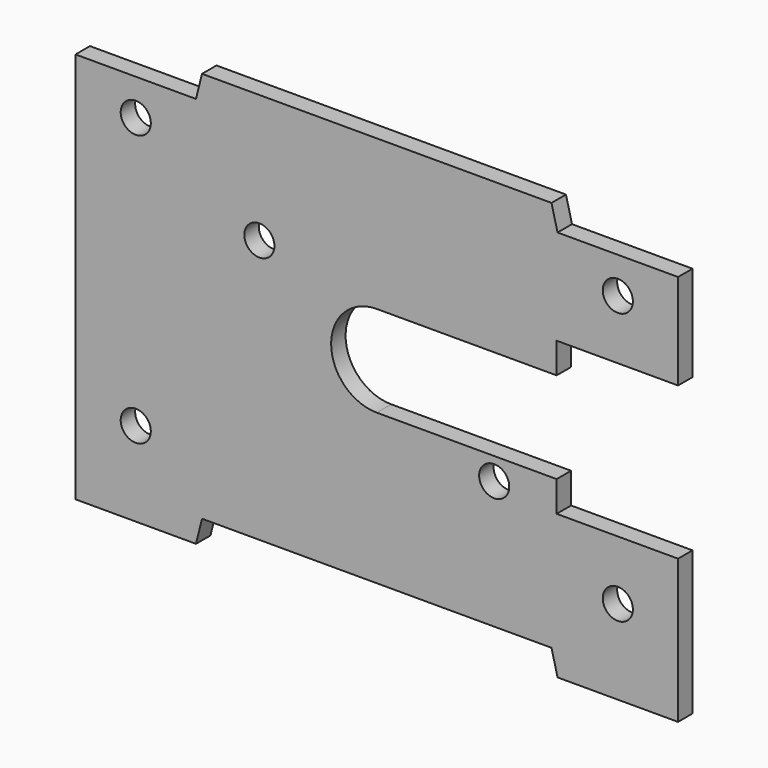
from build123d import *

# Parameters (mm, degrees)
F0_R     = 5
F0_W     = 40
F0_H     = 8
F1_DEPTH = 6


# Not quite as in the source:
# - a feature names something its author has since deleted; it is built from what else it names


with BuildPart() as f1:
    # F0 (on Front) → F1 (new body)
    with BuildSketch(Plane.XZ):
        with BuildLine():
            Line((0, 122), (0, 0))
            Line((0, 0), (40, 0))
            Line((40, 0), (42, 0))
            Line((42, 0), (158, 0))
            Line((158, 0), (160, 0))
            Line((160, 0), (200, 0))
            Line((200, 0), (200, 39.7))
            Line((200, 39.7), (159.7, 39.7))
            Line((159.7, 39.7), (159.7, 49.85))
            Line((159.7, 49.85), (126.2405697347, 49.85))
            Line((126.2405697347, 49.85), (100, 49.85))
            ThreePointArc((100, 49.85), (86.8797151327, 57.425), (86.8797151327, 72.575))
            ThreePointArc((86.8797151327, 72.575), (92.425, 78.1202848673), (100, 80.15))
            Line((100, 80.15), (159.7, 80.15))
            Line((159.7, 80.15), (159.7, 90.3))
            Line((159.7, 90.3), (200, 90.3))
            Line((200, 90.3), (200, 122))
            Line((200, 122), (160, 122))
            Line((160, 122), (158, 130))
            Line((158, 130), (42, 130))
            Line((42, 130), (40, 122))
            Line((40, 122), (0, 122))
        make_face()
        with Locations((20, 20)):
            Circle(F0_R, mode=Mode.SUBTRACT)
        with Locations((180, 20)):
            Circle(F0_R, mode=Mode.SUBTRACT)
        with BuildLine():
            ThreePointArc((143.9711431703, 42.5), (137.6770479448, 37.6703708686), (134.6410161514, 45))
            ThreePointArc((134.6410161514, 45), (140.2652383958, 47.3296291314), (143.9711431703, 42.5))
        make_face(mode=Mode.SUBTRACT)
        with BuildLine():
            ThreePointArc((66.0288568297, 87.5), (65.8584859611, 86.2059047745), (65.3589838486, 85))
            ThreePointArc((65.3589838486, 85), (56.1992276983, 88.7940952255), (66.0288568297, 87.5))
        make_face(mode=Mode.SUBTRACT)
        with Locations((20, 110)):
            Circle(F0_R, mode=Mode.SUBTRACT)
        with Locations((180, 110)):
            Circle(F0_R, mode=Mode.SUBTRACT)
        with Locations((20, -4)):
            Rectangle(F0_W, F0_H)
        with Locations((180, -4)):
            Rectangle(F0_W, F0_H)
        Polygon((42, 0), (40, 0), (40, -8), align=None)
        Polygon((160, 0), (158, 0), (160, -8), align=None)
    extrude(amount=F1_DEPTH)


solid = f1.part
